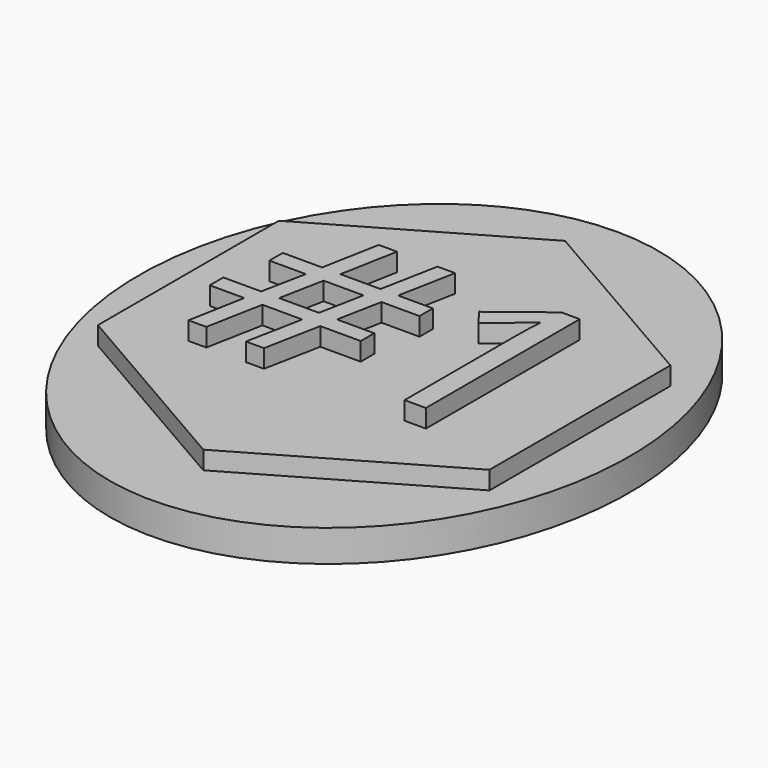
from build123d import *

# Parameters (mm, degrees)
F1_DEPTH     = 4.445
F3_DEPTH     = 2.54
F4_TEXT_SIZE = 37.6539253112
F5_DEPTH     = 2.54


# Not quite as in the source:
# - Text() gives the source's letters only with a copy of the font that has no kerning and outlines rounded to 1/6400 em; it was checked with that copy


with BuildPart() as f1:
    # F0 (on Top) → F1 (new body)
    with BuildSketch(Plane.XY):
        with BuildLine():
            add(Edge.make_bspline(
                [(0, 40.64), (-59.3920221915, 40.64), (-29.6960110958, -20.32), (0, -81.28), (29.6960110958, -20.32), (59.3920221915, 40.64), (0, 40.64)],
                knots=[0, 0, 0, 2.0943951024, 2.0943951024, 4.1887902048, 4.1887902048, 6.2831853072, 6.2831853072, 6.2831853072], degree=2, weights=[1, 0.5, 1, 0.5, 1, 0.5, 1]))
        make_face()
    extrude(amount=F1_DEPTH)

    # F2 (on face) → F3 (join)
    with BuildSketch(Plane.XY.offset(4.445)):
        Polygon((27.3635462546, 15.7983507961), (0, 31.5967015922), (-27.3635462546, 15.7983507961), (-27.3635462546, -15.7983507961), (0, -31.5967015922), (27.3635462546, -15.7983507961), align=None)
    extrude(amount=F3_DEPTH)

    # F4 (on face) → F5 (join)
    with BuildSketch(Plane.XY.offset(6.985)):
        with Locations((-21.6014906764, -12.5414067879)):
            Text('#1', F4_TEXT_SIZE, font='Open Sans', text_align=(TextAlign.LEFT, TextAlign.BOTTOM))
    extrude(amount=F5_DEPTH)


solid = f1.part
